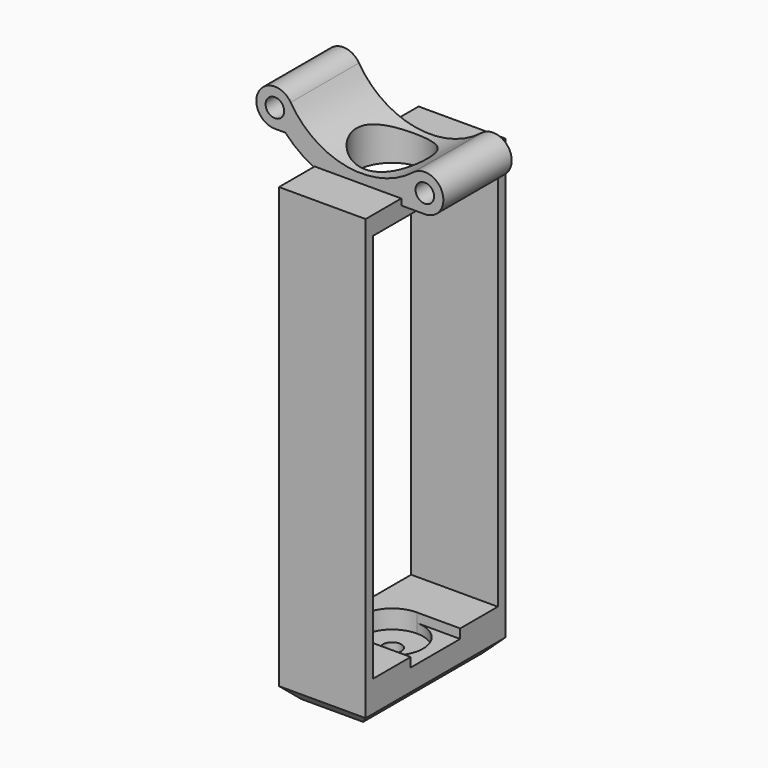
from build123d import *

# Parameters (mm, degrees)
F0_R      = 1.5
F1_DEPTH  = 6.9
F2_W      = 28.2
F2_H      = 73
F2_W_2    = 25.2
F2_H_2    = 63
F3_DEPTH  = 7
F4_R      = 5.75
F5_DEPTH  = 12.2727451706
F6_SIZE   = 2
F7_R      = 1.5
F8_DEPTH  = 3
F9_DEPTH  = 7.001
F10_DEPTH = 1.5


with BuildPart() as f1:
    # F0 (on Front) → F1 (new body, symmetric)
    with BuildSketch(Plane.XZ):
        with BuildLine():
            Line((-7, 2.7587302293), (-7, 0))
            Line((-7, 0), (7, 0))
            Line((7, 0), (7, 2))
            Line((7, 2), (10.8, 2))
            ThreePointArc((10.8, 2), (13.6348625345, 5.9816080739), (8.9448506986, 7.3576303929))
            ThreePointArc((8.9448506986, 7.3576303929), (-1.7475715563, 4.6720624952), (-10.8766435302, 10.8526946234))
            ThreePointArc((-10.8766435302, 10.8526946234), (-16.0476108736, 10.7307091252), (-13.4262707241, 6.2717451706))
            Line((-13.4262707241, 6.2717451706), (-11.7411403572, 6.2717451706))
            ThreePointArc((-11.7411403572, 6.2717451706), (-9.5241596378, 4.3079544417), (-7, 2.7587302293))
        make_face()
        with Locations((10.8, 5)):
            Circle(F0_R, mode=Mode.SUBTRACT)
        with Locations((-13.4262707241, 9.2717451706)):
            Circle(F0_R, mode=Mode.SUBTRACT)
    extrude(amount=F1_DEPTH, both=True)

    # F2 (on Right) → F3 (join, symmetric)
    with BuildSketch(Plane.YZ):
        with Locations((0, -33.5)):
            Rectangle(F2_W, F2_H)
        with Locations((0, -31.5)):
            Rectangle(F2_W_2, F2_H_2, mode=Mode.SUBTRACT)
    extrude(amount=F3_DEPTH, both=True)

    # F4 (on face) → F5 (cut, through all)
    with BuildSketch(Plane(origin=(0, 0, 0), x_dir=(1, 0, 0), z_dir=(0, 0, -1))):
        Circle(F4_R)
    extrude(amount=-F5_DEPTH, mode=Mode.SUBTRACT)

    # F6
    f6_edges = [f1.edges().sort_by_distance(p)[0] for p in [
        (0, -14.1, -70),
        (-7, 0, -70),
        (0, 14.1, -70),
        (7, 0, -70),
    ]]
    chamfer(f6_edges, length=F6_SIZE)

    # F7 (on face) → F8 (cut)
    with BuildSketch(Plane.XY.offset(-63)):
        with BuildLine():
            ThreePointArc((0, -5), (3.5355339059, -3.5355339059), (5, 0))
            ThreePointArc((5, 0), (3.5355339059, 3.5355339059), (0, 5))
            ThreePointArc((0, 5), (-5, 0), (0, -5))
        make_face()
        Circle(F7_R, mode=Mode.SUBTRACT)
    extrude(amount=-F8_DEPTH, mode=Mode.SUBTRACT)

    # F9 (cut, through all): a face of the model
    f9_faces = [f1.faces().sort_by_distance(p)[0] for p in [
        (0, 0, -63),
    ]]
    extrude(f9_faces, amount=-F9_DEPTH, mode=Mode.SUBTRACT)

    # F7 (on face) → F10 (cut)
    with BuildSketch(Plane.XY.offset(-63)):
        with BuildLine():
            ThreePointArc((0, 5), (3.5355339059, 3.5355339059), (5, 0))
            ThreePointArc((5, 0), (3.5355339059, -3.5355339059), (0, -5))
            Line((0, -5), (7, -5))
            Line((7, -5), (7, 5))
            Line((7, 5), (0, 5))
        make_face()
    extrude(amount=-F10_DEPTH, mode=Mode.SUBTRACT)


solid = f1.part
